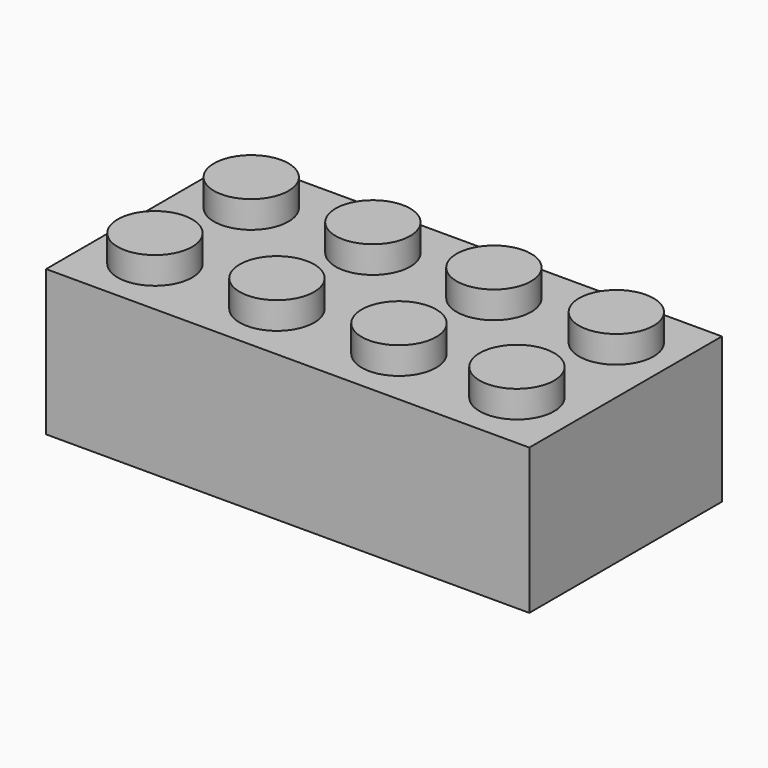
from build123d import *

# Parameters (mm, degrees)
F0_W      = 31.7881
F0_H      = 15.8369
F1_DEPTH  = 4.7879
F2_R      = 2.4511
F3_DEPTH  = 1.778
F4_R      = 2.4511
F5_DEPTH  = 1.778
F6_R      = 2.4511
F7_DEPTH  = 1.778
F8_R      = 2.4511
F9_DEPTH  = 1.778
F10_R     = 2.4511
F11_DEPTH = 1.778
F12_R     = 2.4511
F13_DEPTH = 1.778
F14_R     = 2.4511
F15_DEPTH = 1.778
F16_R     = 2.4511
F17_DEPTH = 1.778
F20_R     = 2.82575
F22_DEPTH = 8.3185
F20_W     = 30.5308
F20_H     = 14.5796
F20_R_2   = 3.2385
F23_DEPTH = 8.3185
F24_R     = 3.2385
F28_DEPTH = 8.3312
F25_R     = 3.2385
F29_DEPTH = 8.3312
F26_R     = 2.8194
F30_DEPTH = 8.3312
F27_R     = 2.8194
F31_DEPTH = 8.3312


# Not quite as in the source:
# - the program builds the solid bodies; features that only make, move or delete a surface that nothing else refers to are left out


with BuildPart() as f1:
    # F0 (on Top) → F1 (new body, symmetric)
    with BuildSketch(Plane.XY):
        Rectangle(F0_W, F0_H)
    extrude(amount=F1_DEPTH, both=True)

    # F2 (on face) → F3 (join)
    with BuildSketch(Plane.XY.offset(4.7879)):
        with Locations((-11.91895, 3.98145)):
            Circle(F2_R)
    extrude(amount=F3_DEPTH)

    # F4 (on face) → F5 (join)
    with BuildSketch(Plane.XY.offset(4.7879)):
        with Locations((-3.9052600634, 3.96875)):
            Circle(F4_R)
    extrude(amount=F5_DEPTH)

    # F6 (on face) → F7 (join)
    with BuildSketch(Plane.XY.offset(4.7879)):
        with Locations((4.0955786651, 3.91795)):
            Circle(F6_R)
    extrude(amount=F7_DEPTH)

    # F8 (on face) → F9 (join)
    with BuildSketch(Plane.XY.offset(4.7879)):
        with Locations((12.096326677, 3.98145)):
            Circle(F8_R)
    extrude(amount=F9_DEPTH)

    # F10 (on face) → F11 (join)
    with BuildSketch(Plane.XY.offset(4.7879)):
        with Locations((-11.89355, -3.96875)):
            Circle(F10_R)
    extrude(amount=F11_DEPTH)

    # F12 (on face) → F13 (join)
    with BuildSketch(Plane.XY.offset(4.7879)):
        with Locations((-3.86715, -3.96875)):
            Circle(F12_R)
    extrude(amount=F13_DEPTH)

    # F14 (on face) → F15 (join)
    with BuildSketch(Plane.XY.offset(4.7879)):
        with Locations((4.15925, -3.96875)):
            Circle(F14_R)
    extrude(amount=F15_DEPTH)

    # F16 (on face) → F17 (join)
    with BuildSketch(Plane.XY.offset(4.7879)):
        with Locations((11.91895, -3.96875)):
            Circle(F16_R)
    extrude(amount=F17_DEPTH)

    # F20 (on face) → F22 (cut)
    with BuildSketch(Plane(origin=(0, 0, -4.7879), x_dir=(1, 0, 0), z_dir=(0, 0, -1))):
        Circle(F20_R)
    extrude(amount=-F22_DEPTH, mode=Mode.SUBTRACT)

    # F20 (on face) → F23 (cut)
    with BuildSketch(Plane(origin=(0, 0, -4.7879), x_dir=(1, 0, 0), z_dir=(0, 0, -1))):
        Rectangle(F20_W, F20_H)
        Circle(F20_R_2, mode=Mode.SUBTRACT)
    extrude(amount=-F23_DEPTH, mode=Mode.SUBTRACT)

    # F24 (on face) → F28 (join)
    with BuildSketch(Plane(origin=(0, 0, -4.7879), x_dir=(1, 0, 0), z_dir=(0, 0, -1))):
        with Locations((-8.4963, 0)):
            Circle(F24_R)
    extrude(amount=-F28_DEPTH)

    # F25 (on face) → F29 (join)
    with BuildSketch(Plane(origin=(0, 0, -4.7879), x_dir=(1, 0, 0), z_dir=(0, 0, -1))):
        with Locations((8.4963, 0)):
            Circle(F25_R)
    extrude(amount=-F29_DEPTH)

    # F26 (on face) → F30 (cut)
    with BuildSketch(Plane(origin=(0, 0, -4.7879), x_dir=(1, 0, 0), z_dir=(0, 0, -1))):
        with Locations((-8.472575021, 0)):
            Circle(F26_R)
    extrude(amount=-F30_DEPTH, mode=Mode.SUBTRACT)

    # F27 (on face) → F31 (cut)
    with BuildSketch(Plane(origin=(0, 0, -4.7879), x_dir=(1, 0, 0), z_dir=(0, 0, -1))):
        with Locations((8.4932660684, 0)):
            Circle(F27_R)
    extrude(amount=-F31_DEPTH, mode=Mode.SUBTRACT)


solid = f1.part
